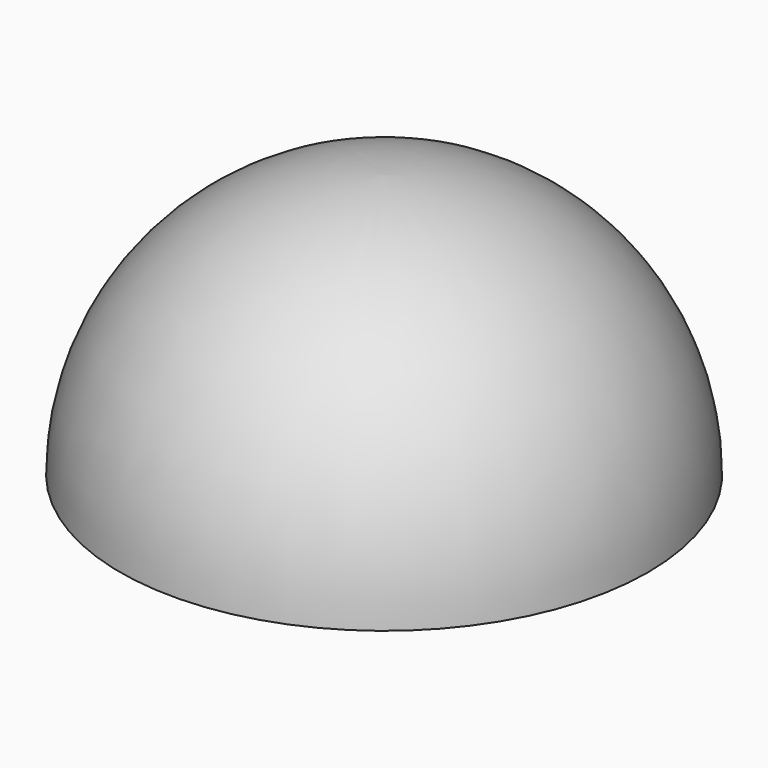
from build123d import *

# Parameters (mm, degrees)
F0_R     = 4
F1_DEPTH = 4
F2_R     = 3.99999


# Not quite as in the source:
# - a fillet or chamfer is up to 0.001 mm smaller than in the source, because OpenCascade refuses the exact size


with BuildPart() as f1:
    # F0 (on Top) → F1 (new body)
    with BuildSketch(Plane.XY):
        Circle(F0_R)
    extrude(amount=F1_DEPTH)

    # F2 (radius 4 in the source; OpenCascade refuses exactly that, so slightly less here)
    f2_edges = [f1.edges().sort_by_distance(p)[0] for p in [
        (-4, 0, 4),
    ]]
    fillet(f2_edges, radius=F2_R)


solid = f1.part
